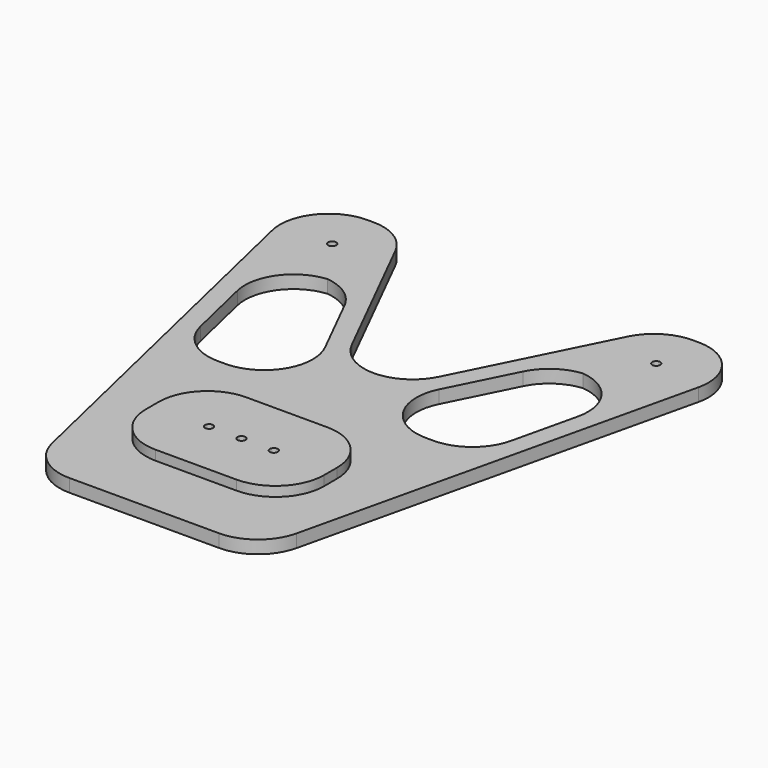
from build123d import *

# Parameters (mm, degrees)
F0_R        = 1.25
F0_W        = 70
F0_H        = 60
F0_W_2      = 55
F0_H_2      = 35
F1_DEPTH    = 4
F2_DEPTH    = 7
F3_T1_DEPTH = 4
F3_T3_DEPTH = 50.3525491562
F3_T5_DEPTH = 98.5146090037
F3_T7_DEPTH = 40.5
F3_T9_DEPTH = 63.5146090037


# Not quite as in the source:
# - a fillet or chamfer that OpenCascade refuses, or shapes differently, is made with other operations: its cross-section is extruded or revolved along the edge and cut away or added


with BuildPart() as f1:
    # F0 (on Top) → F1 (new body)
    with BuildSketch(Plane.XY):
        Polygon((-40, 93.3383707737), (-70, 93.3383707737), (-35, -56.6616292263), (-35, 3.3383707737), (35, 3.3383707737), (35, -56.6616292263), (70, 93.3383707737), (40, 93.3383707737), (0, 13.3383707737), align=None)
        Polygon((-45.172164613, 13.3383707737), (-56.8388312797, 63.3383707737), (-31.7082039325, 63.3383707737), (-6.7082039325, 13.3383707737), align=None, mode=Mode.SUBTRACT)
        with Locations((-50, 78.3383707737)):
            Circle(F0_R, mode=Mode.SUBTRACT)
        Polygon((6.7082039325, 13.3383707737), (31.7082039325, 63.3383707737), (56.8388312797, 63.3383707737), (45.172164613, 13.3383707737), align=None, mode=Mode.SUBTRACT)
        with Locations((50, 78.3383707737)):
            Circle(F0_R, mode=Mode.SUBTRACT)
        with Locations((0, -26.6616292263)):
            Rectangle(F0_W, F0_H)
        with Locations((0, -19.1616292263)):
            Rectangle(F0_W_2, F0_H_2, mode=Mode.SUBTRACT)
        with Locations((0, -19.1616292263)):
            Rectangle(F0_W_2, F0_H_2)
        with Locations((-10, -19.1616292263)):
            Circle(F0_R, mode=Mode.SUBTRACT)
        with Locations((0, -19.1616292263)):
            Circle(F0_R, mode=Mode.SUBTRACT)
        with Locations((10, -19.1616292263)):
            Circle(F0_R, mode=Mode.SUBTRACT)
    extrude(amount=F1_DEPTH)

    # F0 (on Top) → F2 (join)
    with BuildSketch(Plane.XY):
        with Locations((0, -19.1616292263)):
            Rectangle(F0_W_2, F0_H_2)
        with Locations((-10, -19.1616292263)):
            Circle(F0_R, mode=Mode.SUBTRACT)
        with Locations((0, -19.1616292263)):
            Circle(F0_R, mode=Mode.SUBTRACT)
        with Locations((10, -19.1616292263)):
            Circle(F0_R, mode=Mode.SUBTRACT)
    extrude(amount=F2_DEPTH)

    # F3: fillet of radius 15 on 19 edges, made by hand

    # F3_s2 → F3_t1 (join)
    with BuildSketch(Plane.XY):
        with BuildLine():
            ThreePointArc((13.416407865, 40.1711865037), (0, 31.8793904362), (-13.416407865, 40.1711865037))
            Line((-13.416407865, 40.1711865037), (0, 13.3383707737))
            Line((0, 13.3383707737), (13.416407865, 40.1711865037))
        make_face()
        with BuildLine():
            ThreePointArc((17.5623058987, 35.0465747062), (18.2189516385, 20.452404092), (30.9787137637, 13.3383707737))
            Line((30.9787137637, 13.3383707737), (6.7082039325, 13.3383707737))
            Line((6.7082039325, 13.3383707737), (17.5623058987, 35.0465747062))
        make_face()
        with BuildLine():
            ThreePointArc((47.8768609584, 24.9299265396), (42.5932263089, 16.5883353799), (33.2692428123, 13.3383707737))
            Line((33.2692428123, 13.3383707737), (45.172164613, 13.3383707737))
            Line((45.172164613, 13.3383707737), (47.8768609584, 24.9299265396))
        make_face()
        with BuildLine():
            ThreePointArc((-17.5623058987, 35.0465747062), (-18.2189516385, 20.452404092), (-30.9787137637, 13.3383707737))
            Line((-30.9787137637, 13.3383707737), (-6.7082039325, 13.3383707737))
            Line((-6.7082039325, 13.3383707737), (-17.5623058987, 35.0465747062))
        make_face()
        with BuildLine():
            ThreePointArc((-47.8768609584, 24.9299265396), (-42.5932263089, 16.5883353799), (-33.2692428123, 13.3383707737))
            Line((-33.2692428123, 13.3383707737), (-45.172164613, 13.3383707737))
            Line((-45.172164613, 13.3383707737), (-47.8768609584, 24.9299265396))
        make_face()
        with BuildLine():
            ThreePointArc((-37.935909479, 63.3383707737), (-49.6859448728, 57.6623542703), (-52.5435276251, 44.9299265396))
            Line((-52.5435276251, 44.9299265396), (-56.8388312797, 63.3383707737))
            Line((-56.8388312797, 63.3383707737), (-37.935909479, 63.3383707737))
        make_face()
        with BuildLine():
            ThreePointArc((-40.9787137637, 63.3383707737), (-33.092747082, 61.098132899), (-27.5623058987, 55.0465747062))
            Line((-27.5623058987, 55.0465747062), (-31.7082039325, 63.3383707737))
            Line((-31.7082039325, 63.3383707737), (-40.9787137637, 63.3383707737))
        make_face()
        with BuildLine():
            ThreePointArc((40.9787137637, 63.3383707737), (33.092747082, 61.098132899), (27.5623058987, 55.0465747062))
            Line((27.5623058987, 55.0465747062), (31.7082039325, 63.3383707737))
            Line((31.7082039325, 63.3383707737), (40.9787137637, 63.3383707737))
        make_face()
        with BuildLine():
            ThreePointArc((37.935909479, 63.3383707737), (49.6859448728, 57.6623542703), (52.5435276251, 44.9299265396))
            Line((52.5435276251, 44.9299265396), (56.8388312797, 63.3383707737))
            Line((56.8388312797, 63.3383707737), (37.935909479, 63.3383707737))
        make_face()
    extrude(amount=F3_T1_DEPTH)

    # F3_s4 → F3_t3 (cut)
    with BuildSketch(Plane.XY.offset(-23.1762745781)):
        with BuildLine():
            ThreePointArc((49.2705098312, 93.3383707737), (41.3845431495, 91.098132899), (35.8541019662, 85.0465747062))
            Line((35.8541019662, 85.0465747062), (40, 93.3383707737))
            Line((40, 93.3383707737), (49.2705098312, 93.3383707737))
        make_face()
        with BuildLine():
            ThreePointArc((-49.2705098312, 93.3383707737), (-41.3845431495, 91.098132899), (-35.8541019662, 85.0465747062))
            Line((-35.8541019662, 85.0465747062), (-40, 93.3383707737))
            Line((-40, 93.3383707737), (-49.2705098312, 93.3383707737))
        make_face()
    extrude(amount=F3_T3_DEPTH, mode=Mode.SUBTRACT)

    # F3_s6 → F3_t5 (cut)
    with BuildSketch(Plane.XY.offset(-47.2573045019)):
        with BuildLine():
            ThreePointArc((65.7046963454, 74.9299265396), (62.8471135931, 87.6623542703), (51.0970781993, 93.3383707737))
            Line((51.0970781993, 93.3383707737), (70, 93.3383707737))
            Line((70, 93.3383707737), (65.7046963454, 74.9299265396))
        make_face()
        with BuildLine():
            ThreePointArc((-51.0970781993, 93.3383707737), (-62.8471135931, 87.6623542703), (-65.7046963454, 74.9299265396))
            Line((-65.7046963454, 74.9299265396), (-70, 93.3383707737))
            Line((-70, 93.3383707737), (-51.0970781993, 93.3383707737))
        make_face()
    extrude(amount=F3_T5_DEPTH, mode=Mode.SUBTRACT)

    # F3_s8 → F3_t7 (cut)
    with BuildSketch(Plane.XY.offset(4)):
        with BuildLine():
            ThreePointArc((12.5, -1.6616292263), (23.1066017178, -6.0550275085), (27.5, -16.6616292263))
            Line((27.5, -16.6616292263), (27.5, -1.6616292263))
            Line((27.5, -1.6616292263), (12.5, -1.6616292263))
        make_face()
        with BuildLine():
            ThreePointArc((-12.5, -1.6616292263), (-23.1066017178, -6.0550275085), (-27.5, -16.6616292263))
            Line((-27.5, -16.6616292263), (-27.5, -1.6616292263))
            Line((-27.5, -1.6616292263), (-12.5, -1.6616292263))
        make_face()
        with BuildLine():
            ThreePointArc((12.5, -36.6616292263), (23.1066017178, -32.2682309441), (27.5, -21.6616292263))
            Line((27.5, -21.6616292263), (27.5, -36.6616292263))
            Line((27.5, -36.6616292263), (12.5, -36.6616292263))
        make_face()
        with BuildLine():
            ThreePointArc((-27.5, -21.6616292263), (-23.1066017178, -32.2682309441), (-12.5, -36.6616292263))
            Line((-12.5, -36.6616292263), (-27.5, -36.6616292263))
            Line((-27.5, -36.6616292263), (-27.5, -21.6616292263))
        make_face()
    extrude(amount=F3_T7_DEPTH, mode=Mode.SUBTRACT)

    # F3_s10 → F3_t9 (cut)
    with BuildSketch(Plane.XY.offset(-29.7573045019)):
        with BuildLine():
            ThreePointArc((-37.7046963454, -45.0700734604), (-32.4210616958, -53.4116646201), (-23.0970781993, -56.6616292263))
            Line((-23.0970781993, -56.6616292263), (-35, -56.6616292263))
            Line((-35, -56.6616292263), (-37.7046963454, -45.0700734604))
        make_face()
        with BuildLine():
            ThreePointArc((23.0970781993, -56.6616292263), (32.4210616958, -53.4116646201), (37.7046963454, -45.0700734604))
            Line((37.7046963454, -45.0700734604), (35, -56.6616292263))
            Line((35, -56.6616292263), (23.0970781993, -56.6616292263))
        make_face()
    extrude(amount=F3_T9_DEPTH, mode=Mode.SUBTRACT)


solid = f1.part
